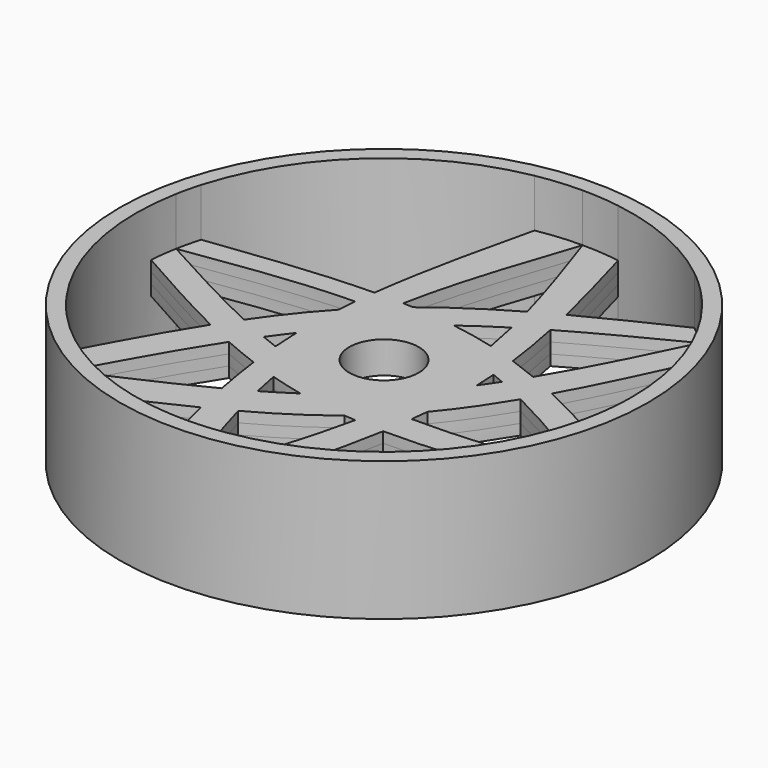
from build123d import *

# Parameters (mm, degrees)
F0_R          = 241.3141538393
F1_DEPTH      = 63.5
F1_DEPTH_BACK = 63.5
F2_DEPTH      = 9.7028
F2_DEPTH_BACK = 9.7028
F3_DEPTH      = 9.7028
F3_DEPTH_BACK = 9.7028
F4_DEPTH      = 9.7028
F4_DEPTH_BACK = 9.7028
F0_R_2        = 31.7673719728
F5_DEPTH      = 9.7028
F5_DEPTH_BACK = 9.7028
F6_DEPTH      = 9.7028
F6_DEPTH_BACK = 9.7028


# Not quite as in the source:
# - a feature of the source that left no trace in its solid (it failed there, or was rolled back) is left out
# - a feature names something its author has since deleted; it is built from what else it names


with BuildPart() as f1:
    # F0 (on Top) → F1 (new body, two sides)
    with BuildSketch(Plane.XY) as f1_sk:
        Circle(F0_R)
        with BuildLine():
            ThreePointArc((178.3079100104, 140.332604898), (214.4135352432, 74.2548764339), (226.9073616472, 0))
            ThreePointArc((226.9073616472, 0), (226.6842601254, -10.0596710247), (226.0153942788, -20.0995601621))
            ThreePointArc((226.0153942788, -20.0995601621), (224.3142281841, -34.2064000428), (221.733453838, -48.1791056247))
            ThreePointArc((221.733453838, -48.1791056247), (218.4875359512, -61.2384471037), (214.4731856165, -74.0824096614))
            ThreePointArc((214.4731856165, -74.0824096614), (145.4794819638, -174.134060704), (34.7509421656, -224.2305126166))
            ThreePointArc((34.7509421656, -224.2305126166), (17.4269439528, -226.2371596228), (0, -226.9073616472))
            ThreePointArc((0, -226.9073616472), (-17.4269439528, -226.2371596228), (-34.7509421656, -224.2305126166))
            ThreePointArc((-34.7509421656, -224.2305126166), (-90.7197460911, -207.9828801581), (-140.7039473309, -178.0150273859))
            ThreePointArc((-140.7039473309, -178.0150273859), (-153.7906323304, -166.8394203332), (-165.9927059169, -154.704144586))
            ThreePointArc((-165.9927059169, -154.704144586), (-176.0017718986, -143.2142697438), (-185.2170956029, -131.0785194688))
            ThreePointArc((-185.2170956029, -131.0785194688), (-218.634724648, -60.7108552716), (-226.2836655529, 16.8123012599))
            ThreePointArc((-226.2836655529, 16.8123012599), (-225.0281851573, 29.1421799891), (-223.1013732807, 41.3851182186))
            ThreePointArc((-223.1013732807, 41.3851182186), (-220.7427090788, 52.5319632059), (-217.8274802779, 63.5463579248))
            ThreePointArc((-217.8274802779, 63.5463579248), (-152.0556560856, 168.4221725964), (-41.0251201184, 223.1678522749))
            ThreePointArc((-41.0251201184, 223.1678522749), (-20.5975994419, 225.9705504417), (0, 226.9073616472))
            ThreePointArc((0, 226.9073616472), (17.325289581, 226.2449670394), (34.5494261777, 224.2616505792))
            ThreePointArc((34.5494261777, 224.2616505792), (91.3796204536, 207.6938028336), (141.9905839779, 176.9904653684))
            ThreePointArc((141.9905839779, 176.9904653684), (151.0506346969, 169.324116792), (159.6974427922, 161.1945332055))
            ThreePointArc((159.6974427922, 161.1945332055), (169.3242736408, 151.050458873), (178.3079100104, 140.332604898))
        make_face(mode=Mode.SUBTRACT)
    extrude(amount=F1_DEPTH)
    extrude(f1_sk.sketch, amount=-F1_DEPTH_BACK)

    # F0 (on Top) → F2 (join, two sides)
    with BuildSketch(Plane.XY) as f2_sk:
        with BuildLine():
            add(Edge.make_bspline(
                [(-223.1013732807, 41.3851182186), (-187.7970771474, 22.1615793919), (-152.5240311166, 2.6878342087), (-116.7614189474, -13.841576746)],
                knots=[0, 0, 0, 0, 0.2511601881, 0.2511601881, 0.2511601881, 0.2511601881], degree=3))
            ThreePointArc((-223.1013732807, 41.3851182186), (-225.0281851573, 29.1421799891), (-226.2836655529, 16.8123012599))
            add(Edge.make_bspline(
                [(-226.2836655529, 16.8123012599), (-194.4717454799, -1.1394771145), (-162.6487337642, -19.090575894), (-130.5710356825, -34.8135274055)],
                knots=[0, 0, 0, 0, 0.2250871065, 0.2250871065, 0.2250871065, 0.2250871065], degree=3))
            add(Edge.make_bspline(
                [(-116.7614189474, -13.841576746), (-121.4836444158, -20.7174022597), (-126.0789503614, -27.7156968125), (-130.5710356828, -34.8135274064)],
                knots=[0.7062454841, 0.7062454841, 0.7062454841, 0.7062454841, 0.7612094599, 0.7612094599, 0.7612094599, 0.7612094599], degree=3))
        make_face()
        with BuildLine():
            ThreePointArc((-185.2170956029, -131.0785194688), (-176.0017718986, -143.2142697438), (-165.9927059169, -154.704144586))
            add(Edge.make_bspline(
                [(-103.8007523743, -47.3412327817), (-126.030548472, -81.5945859435), (-145.9101294083, -118.2760524876), (-165.9927059169, -154.704144586)],
                knots=[0.7370824764, 0.7370824764, 0.7370824764, 0.7370824764, 1, 1, 1, 1], degree=3))
            add(Edge.make_bspline(
                [(-130.5710356825, -34.8135274055), (-121.6689580768, -39.1768995586), (-112.7472657537, -43.3686705384), (-103.8007523743, -47.3412327817)],
                knots=[0.2250871065, 0.2250871065, 0.2250871065, 0.2250871065, 0.2875524021, 0.2875524021, 0.2875524021, 0.2875524021], degree=3))
            add(Edge.make_bspline(
                [(-130.5710356828, -34.8135274064), (-150.0868633876, -65.6499939995), (-167.6544421985, -98.3651644216), (-185.2170956029, -131.0785194688)],
                knots=[0.7612094599, 0.7612094599, 0.7612094599, 0.7612094599, 1, 1, 1, 1], degree=3))
        make_face()
        with BuildLine():
            add(Edge.make_bspline(
                [(-116.7614189474, -13.841576746), (-107.6387205848, -18.0580704836), (-98.4841656138, -22.0829731469), (-89.2891089992, -25.8632585175)],
                knots=[0.2511601881, 0.2511601881, 0.2511601881, 0.2511601881, 0.3152287362, 0.3152287362, 0.3152287362, 0.3152287362], degree=3))
            add(Edge.make_bspline(
                [(-116.7614189474, -13.841576746), (-121.4836444158, -20.7174022597), (-126.0789503614, -27.7156968125), (-130.5710356828, -34.8135274064)],
                knots=[0.7062454841, 0.7062454841, 0.7062454841, 0.7062454841, 0.7612094599, 0.7612094599, 0.7612094599, 0.7612094599], degree=3))
            add(Edge.make_bspline(
                [(-130.5710356825, -34.8135274055), (-121.6689580768, -39.1768995586), (-112.7472657537, -43.3686705384), (-103.8007523743, -47.3412327817)],
                knots=[0.2250871065, 0.2250871065, 0.2250871065, 0.2250871065, 0.2875524021, 0.2875524021, 0.2875524021, 0.2875524021], degree=3))
            add(Edge.make_bspline(
                [(-89.2891089992, -25.8632585175), (-94.2487356362, -32.8958346395), (-99.0777879744, -40.0637315915), (-103.8007523743, -47.3412327817)],
                knots=[0.6812227601, 0.6812227601, 0.6812227601, 0.6812227601, 0.7370824764, 0.7370824764, 0.7370824764, 0.7370824764], degree=3))
        make_face()
        with BuildLine():
            ThreePointArc((-165.9927059169, -154.704144586), (-153.7906323304, -166.8394203332), (-140.7039473309, -178.0150273859))
            add(Edge.make_bspline(
                [(-56.1350371859, -138.940325702), (-83.5712231498, -152.586887822), (-112.1740051357, -165.0586791026), (-140.7039473309, -178.0150273859)],
                knots=[0.8020879998, 0.8020879998, 0.8020879998, 0.8020879998, 1, 1, 1, 1], degree=3))
            add(Edge.make_bspline(
                [(-62.9704662026, -106.5559716315), (-60.8774510593, -117.3512347545), (-58.580284651, -128.146141133), (-56.1350371658, -138.9403257269)],
                knots=[0.7369714232, 0.7369714232, 0.7369714232, 0.7369714232, 0.8093413391, 0.8093413391, 0.8093413391, 0.8093413391], degree=3))
            add(Edge.make_bspline(
                [(-62.9704662042, -106.5559716298), (-95.7578523664, -123.7944289451), (-130.7016529053, -138.8997980839), (-165.9927059169, -154.704144586)],
                knots=[0.7607464131, 0.7607464131, 0.7607464131, 0.7607464131, 1, 1, 1, 1], degree=3))
        make_face()
        with BuildLine():
            add(Edge.make_bspline(
                [(-32.0325540387, -126.4279660664), (-39.9421861303, -130.7313342854), (-47.9871680873, -134.8876340507), (-56.1350371859, -138.940325702)],
                knots=[0.7433130275, 0.7433130275, 0.7433130275, 0.7433130275, 0.8020879998, 0.8020879998, 0.8020879998, 0.8020879998], degree=3))
            add(Edge.make_bspline(
                [(-40.265203536, -94.0296077094), (-37.8015476904, -104.8290604959), (-35.0304565905, -115.6285132824), (-32.0325540365, -126.427966069)],
                knots=[0.7071982306, 0.7071982306, 0.7071982306, 0.7071982306, 0.7785893881, 0.7785893881, 0.7785893881, 0.7785893881], degree=3))
            add(Edge.make_bspline(
                [(-40.2652035459, -94.0296076995), (-47.6992550372, -98.3469624252), (-55.2754717241, -102.5102135071), (-62.9704662042, -106.5559716298)],
                knots=[0.7045950925, 0.7045950925, 0.7045950925, 0.7045950925, 0.7607464131, 0.7607464131, 0.7607464131, 0.7607464131], degree=3))
            add(Edge.make_bspline(
                [(-62.9704662026, -106.5559716315), (-60.8774510593, -117.3512347545), (-58.580284651, -128.146141133), (-56.1350371658, -138.9403257269)],
                knots=[0.7369714232, 0.7369714232, 0.7369714232, 0.7369714232, 0.8093413391, 0.8093413391, 0.8093413391, 0.8093413391], degree=3))
        make_face()
        with BuildLine():
            ThreePointArc((-34.7509421656, -224.2305126166), (-17.4269439528, -226.2371596228), (0, -226.9073616472))
            add(Edge.make_bspline(
                [(-32.0325540365, -126.427966069), (-22.73493984, -159.9210979284), (-11.2557363122, -193.4142297878), (0, -226.9073616472)],
                knots=[0.7785893881, 0.7785893881, 0.7785893881, 0.7785893881, 1, 1, 1, 1], degree=3))
            add(Edge.make_bspline(
                [(-32.0325540387, -126.4279660664), (-39.9421861303, -130.7313342854), (-47.9871680873, -134.8876340507), (-56.1350371859, -138.940325702)],
                knots=[0.7433130275, 0.7433130275, 0.7433130275, 0.7433130275, 0.8020879998, 0.8020879998, 0.8020879998, 0.8020879998], degree=3))
            add(Edge.make_bspline(
                [(-56.1350371658, -138.9403257269), (-49.6930286967, -167.3776225623), (-42.2232488822, -195.8099097806), (-34.7509421656, -224.2305126166)],
                knots=[0.8093413391, 0.8093413391, 0.8093413391, 0.8093413391, 1, 1, 1, 1], degree=3))
        make_face()
        with BuildLine():
            add(Edge.make_bspline(
                [(60.3659257227, -58.8348088049), (58.4669517744, -60.8086435456), (53.2706050834, -66.0612229639), (47.888655793, -71.0891672808), (44.430002216, -74.1731903463)],
                knots=[0.4891405798, 0.4891405798, 0.4891405798, 0.4891405798, 0.5073244479, 0.538264786, 0.538264786, 0.538264786, 0.538264786], degree=3))
            add(Edge.make_bspline(
                [(47.1955269779, -58.2406767098), (51.5760143789, -58.4979061921), (55.9664240103, -58.6943119153), (60.3659257288, -58.8348088167)],
                knots=[0.6237120641, 0.6237120641, 0.6237120641, 0.6237120641, 0.6525763095, 0.6525763095, 0.6525763095, 0.6525763095], degree=3))
            add(Edge.make_bspline(
                [(47.1955269766, -58.2406767095), (46.366376749, -63.5515145884), (45.4413390214, -68.8623524674), (44.430002216, -74.1731903463)],
                knots=[0.6283358025, 0.6283358025, 0.6283358025, 0.6283358025, 0.6634437724, 0.6634437724, 0.6634437724, 0.6634437724], degree=3))
        make_face()
        with BuildLine():
            ThreePointArc((221.733453838, -48.1791056247), (224.3142281841, -34.2064000428), (226.0153942788, -20.0995601621))
            add(Edge.make_bspline(
                [(126.0994867384, 34.1240947789), (160.0186435325, 18.0746130851), (193.0176522959, -1.0122474443), (226.0153942788, -20.0995601621)],
                knots=[0.752086296, 0.752086296, 0.752086296, 0.752086296, 1, 1, 1, 1], degree=3))
            add(Edge.make_bspline(
                [(126.0994867384, 34.1240947789), (122.2078656767, 27.0773550144), (118.2234112411, 20.1283415728), (114.1265769663, 13.3035078657)],
                knots=[0.2438163692, 0.2438163692, 0.2438163692, 0.2438163692, 0.2941816592, 0.2941816592, 0.2941816592, 0.2941816592], degree=3))
            add(Edge.make_bspline(
                [(114.1265769663, 13.3035078657), (150.4723295891, -4.8167201502), (186.0717619128, -26.6529777366), (221.733453838, -48.1791056247)],
                knots=[0.7408189422, 0.7408189422, 0.7408189422, 0.7408189422, 1, 1, 1, 1], degree=3))
        make_face()
        with BuildLine():
            add(Edge.make_bspline(
                [(178.3079100104, 140.332604898), (161.6023122909, 104.6402758365), (144.938669773, 68.2370821736), (126.0994867384, 34.1240947789)],
                knots=[0, 0, 0, 0, 0.2438163692, 0.2438163692, 0.2438163692, 0.2438163692], degree=3))
            ThreePointArc((178.3079100104, 140.332604898), (169.3242736408, 151.050458873), (159.6974427922, 161.1945332055))
            add(Edge.make_bspline(
                [(159.6974427922, 161.1945332055), (140.9740911957, 122.2693377019), (121.7499787846, 82.5474043001), (99.532388565, 45.9349903922)],
                knots=[0, 0, 0, 0, 0.2691785702, 0.2691785702, 0.2691785702, 0.2691785702], degree=3))
            add(Edge.make_bspline(
                [(99.5323885815, 45.9349903786), (108.4605180487, 42.2371577797), (117.3108894654, 38.2825835027), (126.0994867384, 34.1240947789)],
                knots=[0.6878508047, 0.6878508047, 0.6878508047, 0.6878508047, 0.752086296, 0.752086296, 0.752086296, 0.752086296], degree=3))
        make_face()
        with BuildLine():
            add(Edge.make_bspline(
                [(126.0994867384, 34.1240947789), (122.2078656767, 27.0773550144), (118.2234112411, 20.1283415728), (114.1265769663, 13.3035078657)],
                knots=[0.2438163692, 0.2438163692, 0.2438163692, 0.2438163692, 0.2941816592, 0.2941816592, 0.2941816592, 0.2941816592], degree=3))
            add(Edge.make_bspline(
                [(99.5323885815, 45.9349903786), (108.4605180487, 42.2371577797), (117.3108894654, 38.2825835027), (126.0994867384, 34.1240947789)],
                knots=[0.6878508047, 0.6878508047, 0.6878508047, 0.6878508047, 0.752086296, 0.752086296, 0.752086296, 0.752086296], degree=3))
            add(Edge.make_bspline(
                [(99.532388565, 45.9349903922), (95.4389768508, 39.1894485718), (91.243951266, 32.5494596673), (86.9317220877, 26.0394538371)],
                knots=[0.2691785702, 0.2691785702, 0.2691785702, 0.2691785702, 0.3187725497, 0.3187725497, 0.3187725497, 0.3187725497], degree=3))
            add(Edge.make_bspline(
                [(86.9317220877, 26.0394538371), (96.0508128029, 22.0637056796), (105.1116517287, 17.797912), (114.1265769663, 13.3035078657)],
                knots=[0.6765336354, 0.6765336354, 0.6765336354, 0.6765336354, 0.7408189422, 0.7408189422, 0.7408189422, 0.7408189422], degree=3))
        make_face()
        with BuildLine():
            add(Edge.make_bspline(
                [(72.5248897002, -59.0843860265), (71.3623043995, -68.1985786181), (69.9708126845, -77.3125549008), (68.3882994897, -86.4263567185)],
                knots=[0.6317623147, 0.6317623147, 0.6317623147, 0.6317623147, 0.6927246064, 0.6927246064, 0.6927246064, 0.6927246064], degree=3))
            add(Edge.make_bspline(
                [(60.3659257288, -58.8348088167), (64.4114410305, -58.9640012573), (68.4646441716, -59.045919839), (72.5248896994, -59.0843860194)],
                knots=[0.6525763095, 0.6525763095, 0.6525763095, 0.6525763095, 0.6791181212, 0.6791181212, 0.6791181212, 0.6791181212], degree=3))
            add(Edge.make_bspline(
                [(60.3659257227, -58.8348088049), (58.4669517744, -60.8086435456), (53.2706050834, -66.0612229639), (47.888655793, -71.0891672808), (44.430002216, -74.1731903463)],
                knots=[0.4891405798, 0.4891405798, 0.4891405798, 0.4891405798, 0.5073244479, 0.538264786, 0.538264786, 0.538264786, 0.538264786], degree=3))
            add(Edge.make_bspline(
                [(44.430002216, -74.1731903463), (43.7097214036, -77.9556044756), (42.9456663908, -81.7380186049), (42.1413010769, -85.5204327342)],
                knots=[0.6634437724, 0.6634437724, 0.6634437724, 0.6634437724, 0.6884479025, 0.6884479025, 0.6884479025, 0.6884479025], degree=3))
            add(Edge.make_bspline(
                [(42.1413010837, -85.5204327366), (50.8627373609, -86.0716670947), (59.6132744903, -86.3601778015), (68.3882994892, -86.4263567151)],
                knots=[0.6205920902, 0.6205920902, 0.6205920902, 0.6205920902, 0.6790156356, 0.6790156356, 0.6790156356, 0.6790156356], degree=3))
        make_face()
        with BuildLine():
            ThreePointArc((0, -226.9073616472), (17.4269439528, -226.2371596228), (34.7509421656, -224.2305126166))
            add(Edge.make_bspline(
                [(68.3882994897, -86.4263567185), (60.4117725039, -132.36372165), (47.5821906288, -178.2966541593), (34.7509421656, -224.2305126166)],
                knots=[0.6927246064, 0.6927246064, 0.6927246064, 0.6927246064, 1, 1, 1, 1], degree=3))
            add(Edge.make_bspline(
                [(42.1413010837, -85.5204327366), (50.8627373609, -86.0716670947), (59.6132744903, -86.3601778015), (68.3882994892, -86.4263567151)],
                knots=[0.6205920902, 0.6205920902, 0.6205920902, 0.6205920902, 0.6790156356, 0.6790156356, 0.6790156356, 0.6790156356], degree=3))
            add(Edge.make_bspline(
                [(42.1413010769, -85.5204327342), (32.1188887968, -132.6494090385), (15.8382122093, -179.7783853429), (0, -226.9073616472)],
                knots=[0.6884479025, 0.6884479025, 0.6884479025, 0.6884479025, 1, 1, 1, 1], degree=3))
        make_face()
        with BuildLine():
            ThreePointArc((214.4731856165, -74.0824096614), (218.4875359512, -61.2384471037), (221.733453838, -48.1791056247))
            add(Edge.make_bspline(
                [(72.5248896994, -59.0843860194), (121.6119386909, -59.5494296394), (171.7283046479, -53.663459736), (221.733453838, -48.1791056247)],
                knots=[0.6791181212, 0.6791181212, 0.6791181212, 0.6791181212, 1, 1, 1, 1], degree=3))
            add(Edge.make_bspline(
                [(72.5248897002, -59.0843860265), (71.3623043995, -68.1985786181), (69.9708126845, -77.3125549008), (68.3882994897, -86.4263567185)],
                knots=[0.6317623147, 0.6317623147, 0.6317623147, 0.6317623147, 0.6927246064, 0.6927246064, 0.6927246064, 0.6927246064], degree=3))
            add(Edge.make_bspline(
                [(68.3882994892, -86.4263567151), (116.5990987769, -86.78994979), (165.5490656943, -80.4424459657), (214.4731856165, -74.0824096614)],
                knots=[0.6790156356, 0.6790156356, 0.6790156356, 0.6790156356, 1, 1, 1, 1], degree=3))
        make_face()
        with BuildLine():
            add(Edge.make_bspline(
                [(159.6974427922, 161.1945332055), (127.3125749824, 144.6273798519), (94.7583746465, 128.244400412), (63.7576337395, 110.2475227747)],
                knots=[0, 0, 0, 0, 0.2302122603, 0.2302122603, 0.2302122603, 0.2302122603], degree=3))
            ThreePointArc((159.6974427922, 161.1945332055), (151.0506346969, 169.324116792), (141.9905839779, 176.9904653684))
            add(Edge.make_bspline(
                [(141.9905839779, 176.9904653684), (113.68205818, 163.5520272179), (85.3664258812, 150.1027410092), (58.1058267487, 135.6234119333)],
                knots=[0, 0, 0, 0, 0.1962065387, 0.1962065387, 0.1962065387, 0.1962065387], degree=3))
            add(Edge.make_bspline(
                [(58.1058267487, 135.6234119333), (60.1058254664, 127.1652640639), (61.9998462927, 118.7065847162), (63.7576337353, 110.2475227788)],
                knots=[0.1976919219, 0.1976919219, 0.1976919219, 0.1976919219, 0.2542686524, 0.2542686524, 0.2542686524, 0.2542686524], degree=3))
        make_face()
        with BuildLine():
            add(Edge.make_bspline(
                [(63.7576337395, 110.2475227747), (55.6747712661, 105.5551740553), (47.6975141979, 100.7531112553), (39.8563985376, 95.8094640523)],
                knots=[0.2302122603, 0.2302122603, 0.2302122603, 0.2302122603, 0.2902357948, 0.2902357948, 0.2902357948, 0.2902357948], degree=3))
            add(Edge.make_bspline(
                [(58.1058267487, 135.6234119333), (60.1058254664, 127.1652640639), (61.9998462927, 118.7065847162), (63.7576337353, 110.2475227788)],
                knots=[0.1976919219, 0.1976919219, 0.1976919219, 0.1976919219, 0.2542686524, 0.2542686524, 0.2542686524, 0.2542686524], degree=3))
            add(Edge.make_bspline(
                [(58.1058267487, 135.6234119333), (49.7160303444, 131.1672140915), (41.4261644637, 126.6134527547), (33.2671911565, 121.9324177431)],
                knots=[0.1962065387, 0.1962065387, 0.1962065387, 0.1962065387, 0.2565915987, 0.2565915987, 0.2565915987, 0.2565915987], degree=3))
            add(Edge.make_bspline(
                [(33.2671911878, 121.9324177444), (35.6324108412, 113.2247665132), (37.8429009939, 104.517115282), (39.8563985708, 95.8094640508)],
                knots=[0.2313167434, 0.2313167434, 0.2313167434, 0.2313167434, 0.2888797804, 0.2888797804, 0.2888797804, 0.2888797804], degree=3))
        make_face()
        with BuildLine():
            add(Edge.make_bspline(
                [(34.5494261777, 224.2616505792), (42.8349791403, 194.7262948915), (51.1173778447, 165.1780979869), (58.1058267487, 135.6234119333)],
                knots=[0, 0, 0, 0, 0.1976919219, 0.1976919219, 0.1976919219, 0.1976919219], degree=3))
            ThreePointArc((34.5494261777, 224.2616505792), (17.325289581, 226.2449670394), (0, 226.9073616472))
            add(Edge.make_bspline(
                [(0, 226.9073616472), (11.7593291755, 191.9157136796), (23.7625691856, 156.924065712), (33.2671911878, 121.9324177444)],
                knots=[0, 0, 0, 0, 0.2313167434, 0.2313167434, 0.2313167434, 0.2313167434], degree=3))
            add(Edge.make_bspline(
                [(58.1058267487, 135.6234119333), (49.7160303444, 131.1672140915), (41.4261644637, 126.6134527547), (33.2671911565, 121.9324177431)],
                knots=[0.1962065387, 0.1962065387, 0.1962065387, 0.1962065387, 0.2565915987, 0.2565915987, 0.2565915987, 0.2565915987], degree=3))
        make_face()
        with BuildLine():
            add(Edge.make_bspline(
                [(0, 226.9073616472), (-16.8174769673, 176.8644361569), (-34.1338242703, 126.8215106665), (-43.926978592, 76.7785851761)],
                knots=[0, 0, 0, 0, 0.3308151295, 0.3308151295, 0.3308151295, 0.3308151295], degree=3))
            ThreePointArc((0, 226.9073616472), (-20.5975994419, 225.9705504417), (-41.0251201184, 223.1678522749))
            add(Edge.make_bspline(
                [(-41.0251201184, 223.1678522749), (-52.4783431881, 174.4093664115), (-63.9341990007, 125.6686491297), (-70.1940115867, 76.9227656283)],
                knots=[0, 0, 0, 0, 0.32691305, 0.32691305, 0.32691305, 0.32691305], degree=3))
            add(Edge.make_bspline(
                [(-70.1940115868, 76.9227656286), (-61.379684587, 77.0697268961), (-52.6205760006, 77.0328679317), (-43.926978593, 76.7785851835)],
                knots=[0.3061572354, 0.3061572354, 0.3061572354, 0.3061572354, 0.3622331035, 0.3622331035, 0.3622331035, 0.3622331035], degree=3))
        make_face()
        with BuildLine():
            add(Edge.make_bspline(
                [(-43.926978592, 76.7785851761), (-44.5432752393, 73.6293151671), (-45.1297773513, 70.480045158), (-45.6844855831, 67.330775149)],
                knots=[0.3308151295, 0.3308151295, 0.3308151295, 0.3308151295, 0.3516337798, 0.3516337798, 0.3516337798, 0.3516337798], degree=3))
            add(Edge.make_bspline(
                [(-70.1940115868, 76.9227656286), (-61.379684587, 77.0697268961), (-52.6205760006, 77.0328679317), (-43.926978593, 76.7785851835)],
                knots=[0.3061572354, 0.3061572354, 0.3061572354, 0.3061572354, 0.3622331035, 0.3622331035, 0.3622331035, 0.3622331035], degree=3))
            add(Edge.make_bspline(
                [(-70.1940115867, 76.9227656283), (-71.0199395156, 70.4911694667), (-71.7554120654, 64.0594833688), (-72.3884883871, 57.6276546558)],
                knots=[0.32691305, 0.32691305, 0.32691305, 0.32691305, 0.370046389, 0.370046389, 0.370046389, 0.370046389], degree=3))
            add(Edge.make_bspline(
                [(-72.3884883872, 57.6276546558), (-67.0646442905, 57.7244107708), (-61.7571998837, 57.7395100868), (-56.468043341, 57.6635508246)],
                knots=[0.3185902737, 0.3185902737, 0.3185902737, 0.3185902737, 0.3529732947, 0.3529732947, 0.3529732947, 0.3529732947], degree=3))
            add(Edge.make_bspline(
                [(-45.6844855556, 67.3307751349), (-49.3482288534, 64.1752671457), (-52.9443087815, 60.9543566074), (-56.4680433413, 57.6635508256)],
                knots=[0.4662407645, 0.4662407645, 0.4662407645, 0.4662407645, 0.4984116757, 0.4984116757, 0.4984116757, 0.4984116757], degree=3))
        make_face()
        with BuildLine():
            add(Edge.make_bspline(
                [(-217.8274802779, 63.5463579248), (-168.0870830213, 69.8386711876), (-118.3175641023, 76.1204016734), (-70.1940115868, 76.9227656286)],
                knots=[0, 0, 0, 0, 0.3061572354, 0.3061572354, 0.3061572354, 0.3061572354], degree=3))
            ThreePointArc((-217.8274802779, 63.5463579248), (-220.7427090788, 52.5319632059), (-223.1013732807, 41.3851182186))
            add(Edge.make_bspline(
                [(-223.1013732807, 41.3851182186), (-172.457132659, 48.8237580971), (-121.7187944055, 56.7311203711), (-72.3884883872, 57.6276546558)],
                knots=[0, 0, 0, 0, 0.3185902737, 0.3185902737, 0.3185902737, 0.3185902737], degree=3))
            add(Edge.make_bspline(
                [(-70.1940115867, 76.9227656283), (-71.0199395156, 70.4911694667), (-71.7554120654, 64.0594833688), (-72.3884883871, 57.6276546558)],
                knots=[0.32691305, 0.32691305, 0.32691305, 0.32691305, 0.370046389, 0.370046389, 0.370046389, 0.370046389], degree=3))
        make_face()
        with BuildLine():
            add(Edge.make_bspline(
                [(-45.6844855831, 67.330775149), (-46.2652649637, 64.0334902339), (-46.8111916233, 60.7362053189), (-47.3199708539, 57.4389204039)],
                knots=[0.3516337798, 0.3516337798, 0.3516337798, 0.3516337798, 0.3734309015, 0.3734309015, 0.3734309015, 0.3734309015], degree=3))
            add(Edge.make_bspline(
                [(-45.6844855556, 67.3307751349), (-49.3482288534, 64.1752671457), (-52.9443087815, 60.9543566074), (-56.4680433413, 57.6635508256)],
                knots=[0.4662407645, 0.4662407645, 0.4662407645, 0.4662407645, 0.4984116757, 0.4984116757, 0.4984116757, 0.4984116757], degree=3))
            add(Edge.make_bspline(
                [(-56.468043341, 57.6635508246), (-53.412461006, 57.6196686332), (-50.3629821594, 57.5453960707), (-47.3199708543, 57.4389204085)],
                knots=[0.3529732947, 0.3529732947, 0.3529732947, 0.3529732947, 0.3728366038, 0.3728366038, 0.3728366038, 0.3728366038], degree=3))
        make_face()
        with BuildLine():
            add(Edge.make_bspline(
                [(-74.8748334574, -6.3317792212), (-79.8096642217, -12.7072810815), (-84.6075579763, -19.2249838353), (-89.2891089992, -25.8632585175)],
                knots=[0.6284949781, 0.6284949781, 0.6284949781, 0.6284949781, 0.6812227601, 0.6812227601, 0.6812227601, 0.6812227601], degree=3))
            add(Edge.make_bspline(
                [(-73.8401592874, 40.262906217), (-74.7563166341, 26.8429241355), (-75.2465760161, 11.3117584788), (-74.9320157638, -4.2211556835), (-74.8748334608, -6.3317792203)],
                knots=[0.4088628756, 0.4088628756, 0.4088628756, 0.4088628756, 0.4988562077, 0.5130072176, 0.5130072176, 0.5130072176, 0.5130072176], degree=3))
            add(Edge.make_bspline(
                [(-73.8401592874, 40.262906217), (-89.4730644421, 23.5083445643), (-103.6094896571, 5.3083710008), (-116.7614189474, -13.841576746)],
                knots=[0.553164627, 0.553164627, 0.553164627, 0.553164627, 0.7062454841, 0.7062454841, 0.7062454841, 0.7062454841], degree=3))
            add(Edge.make_bspline(
                [(-116.7614189474, -13.841576746), (-107.6387205848, -18.0580704836), (-98.4841656138, -22.0829731469), (-89.2891089992, -25.8632585175)],
                knots=[0.2511601881, 0.2511601881, 0.2511601881, 0.2511601881, 0.3152287362, 0.3152287362, 0.3152287362, 0.3152287362], degree=3))
        make_face()
        with BuildLine():
            add(Edge.make_bspline(
                [(39.8563985376, 95.8094640523), (28.1496006924, 88.4285911089), (16.7462693467, 80.7321189379), (5.7480277227, 72.6139837278)],
                knots=[0.2902357948, 0.2902357948, 0.2902357948, 0.2902357948, 0.3798510249, 0.3798510249, 0.3798510249, 0.3798510249], degree=3))
            add(Edge.make_bspline(
                [(33.2671911878, 121.9324177444), (35.6324108412, 113.2247665132), (37.8429009939, 104.517115282), (39.8563985708, 95.8094640508)],
                knots=[0.2313167434, 0.2313167434, 0.2313167434, 0.2313167434, 0.2888797804, 0.2888797804, 0.2888797804, 0.2888797804], degree=3))
            add(Edge.make_bspline(
                [(33.2671911565, 121.9324177431), (9.2009096149, 108.1249076248), (-13.7265338796, 93.2100458867), (-34.7205364248, 76.425357331)],
                knots=[0.2565915987, 0.2565915987, 0.2565915987, 0.2565915987, 0.4347076189, 0.4347076189, 0.4347076189, 0.4347076189], degree=3))
            add(Edge.make_bspline(
                [(-34.7205364244, 76.4253573294), (-21.0444056104, 75.7730059641), (-7.5413053085, 74.5468801984), (5.7480277227, 72.6139837278)],
                knots=[0.3820816414, 0.3820816414, 0.3820816414, 0.3820816414, 0.4707824274, 0.4707824274, 0.4707824274, 0.4707824274], degree=3))
        make_face()
        with BuildLine():
            add(Edge.make_bspline(
                [(-40.265203536, -94.0296077094), (-37.8015476904, -104.8290604959), (-35.0304565905, -115.6285132824), (-32.0325540365, -126.427966069)],
                knots=[0.7071982306, 0.7071982306, 0.7071982306, 0.7071982306, 0.7785893881, 0.7785893881, 0.7785893881, 0.7785893881], degree=3))
            add(Edge.make_bspline(
                [(31.9130911216, -84.7499075032), (12.2215313381, -100.5355617573), (-9.3489145049, -114.0865508996), (-32.0325540387, -126.4279660664)],
                knots=[0.5747552146, 0.5747552146, 0.5747552146, 0.5747552146, 0.7433130275, 0.7433130275, 0.7433130275, 0.7433130275], degree=3))
            add(Edge.make_bspline(
                [(-14.2194983817, -77.7999720616), (-11.9253735013, -78.3022354633), (3.3554365238, -81.4870898234), (18.7563063515, -83.5956084544), (31.9130911219, -84.7499075041)],
                knots=[0.4937168769, 0.4937168769, 0.4937168769, 0.4937168769, 0.5093492669, 0.597722539, 0.597722539, 0.597722539, 0.597722539], degree=3))
            add(Edge.make_bspline(
                [(-14.2194983817, -77.7999720616), (-22.6709402637, -83.4725390625), (-31.3662142842, -88.8614845856), (-40.2652035459, -94.0296076995)],
                knots=[0.6373787168, 0.6373787168, 0.6373787168, 0.6373787168, 0.7045950925, 0.7045950925, 0.7045950925, 0.7045950925], degree=3))
        make_face()
        with BuildLine():
            add(Edge.make_bspline(
                [(114.1265769663, 13.3035078657), (102.0034881539, -6.892101625), (88.8963470271, -26.0003332005), (74.2986728866, -43.3357359438)],
                knots=[0.2941816592, 0.2941816592, 0.2941816592, 0.2941816592, 0.4432193901, 0.4432193901, 0.4432193901, 0.4432193901], degree=3))
            add(Edge.make_bspline(
                [(86.9317220877, 26.0394538371), (96.0508128029, 22.0637056796), (105.1116517287, 17.797912), (114.1265769663, 13.3035078657)],
                knots=[0.6765336354, 0.6765336354, 0.6765336354, 0.6765336354, 0.7408189422, 0.7408189422, 0.7408189422, 0.7408189422], degree=3))
            add(Edge.make_bspline(
                [(86.9317220877, 26.0394538371), (83.4755802865, 20.8218500539), (79.9441514206, 15.6877423806), (76.3294093346, 10.6497083496)],
                knots=[0.3187725497, 0.3187725497, 0.3187725497, 0.3187725497, 0.3585208604, 0.3585208604, 0.3585208604, 0.3585208604], degree=3))
            add(Edge.make_bspline(
                [(76.3294093346, 10.6497083496), (76.4228091123, 7.0997663821), (76.6686957813, -10.8962895344), (75.7033319421, -28.8911499579), (74.2986728866, -43.3357359438)],
                knots=[0.4762959402, 0.4762959402, 0.4762959402, 0.4762959402, 0.5000370192, 0.5966500368, 0.5966500368, 0.5966500368, 0.5966500368], degree=3))
        make_face()
        with BuildLine():
            add(Edge.make_bspline(
                [(63.7576337353, 110.2475227788), (67.5092172163, 92.1936464903), (70.6402460129, 74.1380274734), (72.8565835725, 56.0821131885)],
                knots=[0.2542686524, 0.2542686524, 0.2542686524, 0.2542686524, 0.3750183644, 0.3750183644, 0.3750183644, 0.3750183644], degree=3))
            add(Edge.make_bspline(
                [(63.7576337395, 110.2475227747), (55.6747712661, 105.5551740553), (47.6975141979, 100.7531112553), (39.8563985376, 95.8094640523)],
                knots=[0.2302122603, 0.2302122603, 0.2302122603, 0.2302122603, 0.2902357948, 0.2902357948, 0.2902357948, 0.2902357948], degree=3))
            add(Edge.make_bspline(
                [(39.8563985708, 95.8094640508), (42.2874442267, 85.2960678886), (44.4313233221, 74.7826717265), (46.2136505599, 64.2692755643)],
                knots=[0.2888797804, 0.2888797804, 0.2888797804, 0.2888797804, 0.3583799241, 0.3583799241, 0.3583799241, 0.3583799241], degree=3))
            add(Edge.make_bspline(
                [(46.2136505599, 64.2692755643), (55.1915373321, 61.8602745475), (64.0677105755, 59.1153416619), (72.8565835745, 56.0821131912)],
                knots=[0.5623988795, 0.5623988795, 0.5623988795, 0.5623988795, 0.6244574438, 0.6244574438, 0.6244574438, 0.6244574438], degree=3))
        make_face()
        with BuildLine():
            add(Edge.make_bspline(
                [(-40.2652035459, -94.0296076995), (-47.6992550372, -98.3469624252), (-55.2754717241, -102.5102135071), (-62.9704662042, -106.5559716298)],
                knots=[0.7045950925, 0.7045950925, 0.7045950925, 0.7045950925, 0.7607464131, 0.7607464131, 0.7607464131, 0.7607464131], degree=3))
            add(Edge.make_bspline(
                [(-45.282922279, -69.5800492168), (-43.8085348876, -77.7299020476), (-42.1244118649, -85.8797548785), (-40.265203536, -94.0296077094)],
                knots=[0.653322591, 0.653322591, 0.653322591, 0.653322591, 0.7071982306, 0.7071982306, 0.7071982306, 0.7071982306], degree=3))
            add(Edge.make_bspline(
                [(-70.4345665727, -61.0026125154), (-62.0789232061, -64.1133073799), (-53.6964231494, -66.9850844484), (-45.282922279, -69.5800492168)],
                knots=[0.3649186891, 0.3649186891, 0.3649186891, 0.3649186891, 0.4228089569, 0.4228089569, 0.4228089569, 0.4228089569], degree=3))
            add(Edge.make_bspline(
                [(-70.4345665657, -61.0026125069), (-68.4544405797, -76.1870941285), (-65.9143983038, -91.371885769), (-62.9704662026, -106.5559716315)],
                knots=[0.6351794609, 0.6351794609, 0.6351794609, 0.6351794609, 0.7369714232, 0.7369714232, 0.7369714232, 0.7369714232], degree=3))
        make_face()
        with BuildLine():
            add(Edge.make_bspline(
                [(-73.4881541081, -32.0929897185), (-72.7224001604, -41.7292326761), (-71.6912432322, -51.3658601577), (-70.4345665657, -61.0026125069)],
                knots=[0.570577721, 0.570577721, 0.570577721, 0.570577721, 0.6351794609, 0.6351794609, 0.6351794609, 0.6351794609], degree=3))
            add(Edge.make_bspline(
                [(-89.2891089992, -25.8632585175), (-84.0358809303, -28.0229734654), (-78.7694333213, -30.1028465153), (-73.4881541081, -32.0929897185)],
                knots=[0.3152287362, 0.3152287362, 0.3152287362, 0.3152287362, 0.3518317403, 0.3518317403, 0.3518317403, 0.3518317403], degree=3))
            add(Edge.make_bspline(
                [(-89.2891089992, -25.8632585175), (-94.2487356362, -32.8958346395), (-99.0777879744, -40.0637315915), (-103.8007523743, -47.3412327817)],
                knots=[0.6812227601, 0.6812227601, 0.6812227601, 0.6812227601, 0.7370824764, 0.7370824764, 0.7370824764, 0.7370824764], degree=3))
            add(Edge.make_bspline(
                [(-103.8007523743, -47.3412327817), (-92.720063225, -52.2614430892), (-81.6012985272, -56.8453867675), (-70.4345665727, -61.0026125154)],
                knots=[0.2875524021, 0.2875524021, 0.2875524021, 0.2875524021, 0.3649186891, 0.3649186891, 0.3649186891, 0.3649186891], degree=3))
        make_face()
        with BuildLine():
            add(Edge.make_bspline(
                [(99.532388565, 45.9349903922), (95.4389768508, 39.1894485718), (91.243951266, 32.5494596673), (86.9317220877, 26.0394538371)],
                knots=[0.2691785702, 0.2691785702, 0.2691785702, 0.2691785702, 0.3187725497, 0.3187725497, 0.3187725497, 0.3187725497], degree=3))
            add(Edge.make_bspline(
                [(72.8565835745, 56.0821131912), (81.8344934769, 52.983644033), (90.7213073249, 49.5843442126), (99.5323885815, 45.9349903786)],
                knots=[0.6244574438, 0.6244574438, 0.6244574438, 0.6244574438, 0.6878508047, 0.6878508047, 0.6878508047, 0.6878508047], degree=3))
            add(Edge.make_bspline(
                [(72.8565835725, 56.0821131885), (73.8858717177, 47.6967756554), (74.7178827755, 39.31137444), (75.3231554266, 30.926054523)],
                knots=[0.3750183644, 0.3750183644, 0.3750183644, 0.3750183644, 0.4310956739, 0.4310956739, 0.4310956739, 0.4310956739], degree=3))
            add(Edge.make_bspline(
                [(75.3231554265, 30.926054523), (79.20373141, 29.3522262649), (83.0729420123, 27.7218077311), (86.9317220877, 26.0394538371)],
                knots=[0.6493310481, 0.6493310481, 0.6493310481, 0.6493310481, 0.6765336354, 0.6765336354, 0.6765336354, 0.6765336354], degree=3))
        make_face()
        with BuildLine():
            add(Edge.make_bspline(
                [(-72.3884883872, 57.6276546558), (-67.0646442905, 57.7244107708), (-61.7571998837, 57.7395100868), (-56.468043341, 57.6635508246)],
                knots=[0.3185902737, 0.3185902737, 0.3185902737, 0.3185902737, 0.3529732947, 0.3529732947, 0.3529732947, 0.3529732947], degree=3))
            add(Edge.make_bspline(
                [(-72.3884883871, 57.6276546558), (-72.9582054354, 51.8395334711), (-73.4449965729, 46.051296789), (-73.8401592874, 40.262906217)],
                knots=[0.370046389, 0.370046389, 0.370046389, 0.370046389, 0.4088628756, 0.4088628756, 0.4088628756, 0.4088628756], degree=3))
            add(Edge.make_bspline(
                [(-56.4680433413, 57.6635508256), (-57.1536029669, 57.0233086218), (-63.1268317058, 51.3994118216), (-68.8878664111, 45.5705246986), (-73.8401592874, 40.262906217)],
                knots=[0.4984116757, 0.4984116757, 0.4984116757, 0.4984116757, 0.5046706823, 0.553164627, 0.553164627, 0.553164627, 0.553164627], degree=3))
        make_face()
        with BuildLine():
            add(Edge.make_bspline(
                [(-43.926978593, 76.7785851835), (-40.8498047075, 76.6885796087), (-37.7808385026, 76.5713337219), (-34.7205364244, 76.4253573294)],
                knots=[0.3622331035, 0.3622331035, 0.3622331035, 0.3622331035, 0.3820816414, 0.3820816414, 0.3820816414, 0.3820816414], degree=3))
            add(Edge.make_bspline(
                [(-43.926978592, 76.7785851761), (-44.5432752393, 73.6293151671), (-45.1297773513, 70.480045158), (-45.6844855831, 67.330775149)],
                knots=[0.3308151295, 0.3308151295, 0.3308151295, 0.3308151295, 0.3516337798, 0.3516337798, 0.3516337798, 0.3516337798], degree=3))
            add(Edge.make_bspline(
                [(-34.7205364248, 76.425357331), (-38.4372539863, 73.453844558), (-42.0933733733, 70.4237274135), (-45.6844855556, 67.3307751349)],
                knots=[0.4347076189, 0.4347076189, 0.4347076189, 0.4347076189, 0.4662407645, 0.4662407645, 0.4662407645, 0.4662407645], degree=3))
        make_face()
        with BuildLine():
            add(Edge.make_bspline(
                [(31.9130911219, -84.7499075041), (35.3178509045, -85.0486211375), (38.7273464546, -85.3046553087), (42.1413010837, -85.5204327366)],
                knots=[0.597722539, 0.597722539, 0.597722539, 0.597722539, 0.6205920902, 0.6205920902, 0.6205920902, 0.6205920902], degree=3))
            add(Edge.make_bspline(
                [(44.430002216, -74.1731903463), (43.7097214036, -77.9556044756), (42.9456663908, -81.7380186049), (42.1413010769, -85.5204327342)],
                knots=[0.6634437724, 0.6634437724, 0.6634437724, 0.6634437724, 0.6884479025, 0.6884479025, 0.6884479025, 0.6884479025], degree=3))
            add(Edge.make_bspline(
                [(44.430002216, -74.1731903463), (40.3509339395, -77.8104267362), (36.1760406973, -81.3325323005), (31.9130911216, -84.7499075032)],
                knots=[0.538264786, 0.538264786, 0.538264786, 0.538264786, 0.5747552146, 0.5747552146, 0.5747552146, 0.5747552146], degree=3))
        make_face()
        with BuildLine():
            add(Edge.make_bspline(
                [(60.3659257288, -58.8348088167), (64.4114410305, -58.9640012573), (68.4646441716, -59.045919839), (72.5248896994, -59.0843860194)],
                knots=[0.6525763095, 0.6525763095, 0.6525763095, 0.6525763095, 0.6791181212, 0.6791181212, 0.6791181212, 0.6791181212], degree=3))
            add(Edge.make_bspline(
                [(74.2986728866, -43.3357359438), (73.788174609, -48.5853630594), (73.1945006518, -53.8349104219), (72.5248897002, -59.0843860265)],
                knots=[0.5966500368, 0.5966500368, 0.5966500368, 0.5966500368, 0.6317623147, 0.6317623147, 0.6317623147, 0.6317623147], degree=3))
            add(Edge.make_bspline(
                [(74.2986728866, -43.3357359438), (69.8008684792, -48.6770834839), (65.1615578938, -53.8501246328), (60.3659257227, -58.8348088049)],
                knots=[0.4432193901, 0.4432193901, 0.4432193901, 0.4432193901, 0.4891405798, 0.4891405798, 0.4891405798, 0.4891405798], degree=3))
        make_face()
    extrude(amount=F2_DEPTH)
    extrude(f2_sk.sketch, amount=-F2_DEPTH_BACK)

    # F0 (on Top) → F2, piece 2 (join, two sides)
    with BuildSketch(Plane.XY) as f2_2_sk:
        with BuildLine():
            add(Edge.make_bspline(
                [(15.994177773, -55.2903259997), (6.3480987535, -63.3085225022), (-3.7485580572, -70.7719274531), (-14.2194983817, -77.7999720616)],
                knots=[0.554100778, 0.554100778, 0.554100778, 0.554100778, 0.6373787168, 0.6373787168, 0.6373787168, 0.6373787168], degree=3))
            add(Edge.make_bspline(
                [(-49.6052252782, -40.4132889191), (-35.51325606, -44.9045731385), (-13.7769520223, -50.6552663039), (8.311170121, -54.2683340591), (15.9941777688, -55.2903259887)],
                knots=[0.4067628451, 0.4067628451, 0.4067628451, 0.4067628451, 0.5035478242, 0.5547829392, 0.5547829392, 0.5547829392, 0.5547829392], degree=3))
            add(Edge.make_bspline(
                [(-49.6052253017, -40.4132889297), (-48.5021480506, -50.1355423587), (-47.0417721834, -59.8577957877), (-45.282922279, -69.5800492168)],
                knots=[0.5890523971, 0.5890523971, 0.5890523971, 0.5890523971, 0.653322591, 0.653322591, 0.653322591, 0.653322591], degree=3))
            add(Edge.make_bspline(
                [(-45.282922279, -69.5800492168), (-34.9774967065, -72.7585377789), (-24.6255605847, -75.5217245937), (-14.2194983817, -77.7999720616)],
                knots=[0.4228089569, 0.4228089569, 0.4228089569, 0.4228089569, 0.4937168769, 0.4937168769, 0.4937168769, 0.4937168769], degree=3))
        make_face()
    extrude(amount=F2_DEPTH)
    extrude(f2_2_sk.sketch, amount=-F2_DEPTH_BACK)

    # F0 (on Top) → F2, piece 3 (join, two sides)
    with BuildSketch(Plane.XY) as f2_3_sk:
        with BuildLine():
            add(Edge.make_bspline(
                [(15.9941777688, -55.2903259887), (26.3305065582, -56.6652620929), (36.7347247171, -57.626401059), (47.1955269779, -58.2406767098)],
                knots=[0.5547829392, 0.5547829392, 0.5547829392, 0.5547829392, 0.6237120641, 0.6237120641, 0.6237120641, 0.6237120641], degree=3))
            add(Edge.make_bspline(
                [(51.3212515182, -20.9088102779), (50.5546869972, -33.3527657551), (49.1383293652, -45.7967212323), (47.1955269766, -58.2406767095)],
                knots=[0.5460734507, 0.5460734507, 0.5460734507, 0.5460734507, 0.6283358025, 0.6283358025, 0.6283358025, 0.6283358025], degree=3))
            add(Edge.make_bspline(
                [(51.3212515182, -20.9088102779), (45.3051450655, -27.7329701051), (33.914203461, -39.6800411725), (21.6803851525, -50.5637290031), (15.994177773, -55.2903259997)],
                knots=[0.4454913911, 0.4454913911, 0.4454913911, 0.4454913911, 0.5050097816, 0.554100778, 0.554100778, 0.554100778, 0.554100778], degree=3))
        make_face()
    extrude(amount=F2_DEPTH)
    extrude(f2_3_sk.sketch, amount=-F2_DEPTH_BACK)

    # F0 (on Top) → F2, piece 4 (join, two sides)
    with BuildSketch(Plane.XY) as f2_4_sk:
        with BuildLine():
            add(Edge.make_bspline(
                [(75.3231554266, 30.926054523), (75.8110262845, 24.1671943387), (76.1515869684, 17.4083869734), (76.3294093346, 10.6497083496)],
                knots=[0.4310956739, 0.4310956739, 0.4310956739, 0.4310956739, 0.4762959402, 0.4762959402, 0.4762959402, 0.4762959402], degree=3))
            add(Edge.make_bspline(
                [(49.6045199666, 40.4195051352), (58.2387027196, 37.5602673322), (66.8082891483, 34.3793916613), (75.3231554265, 30.926054523)],
                knots=[0.5896423849, 0.5896423849, 0.5896423849, 0.5896423849, 0.6493310481, 0.6493310481, 0.6493310481, 0.6493310481], degree=3))
            add(Edge.make_bspline(
                [(49.6045199682, 40.4195051375), (51.133383371, 26.9463367583), (52.4120219557, 6.5035649532), (51.7505885342, -13.9392068519), (51.3212515182, -20.9088102779)],
                knots=[0.4109339053, 0.4109339053, 0.4109339053, 0.4109339053, 0.5, 0.5460734507, 0.5460734507, 0.5460734507, 0.5460734507], degree=3))
            add(Edge.make_bspline(
                [(76.3294093346, 10.6497083496), (68.4202420907, -0.3736655965), (60.1122145505, -10.9370889927), (51.3212515182, -20.9088102779)],
                knots=[0.3585208604, 0.3585208604, 0.3585208604, 0.3585208604, 0.4454913911, 0.4454913911, 0.4454913911, 0.4454913911], degree=3))
        make_face()
    extrude(amount=F2_DEPTH)
    extrude(f2_4_sk.sketch, amount=-F2_DEPTH_BACK)

    # F0 (on Top) → F3 (join, two sides)
    with BuildSketch(Plane.XY) as f3_sk:
        with BuildLine():
            add(Edge.make_bspline(
                [(-51.2671708451, 21.7699117997), (-59.5036240987, 12.7846051269), (-67.3484915269, 3.391797791), (-74.8748334574, -6.3317792212)],
                knots=[0.5480773639, 0.5480773639, 0.5480773639, 0.5480773639, 0.6284949781, 0.6284949781, 0.6284949781, 0.6284949781], degree=3))
            add(Edge.make_bspline(
                [(-47.3199708539, 57.4389204039), (-49.1545763167, 45.5492508699), (-50.5061726075, 33.659581336), (-51.2671708513, 21.769911802)],
                knots=[0.3734309015, 0.3734309015, 0.3734309015, 0.3734309015, 0.4520290756, 0.4520290756, 0.4520290756, 0.4520290756], degree=3))
            add(Edge.make_bspline(
                [(-56.468043341, 57.6635508246), (-53.412461006, 57.6196686332), (-50.3629821594, 57.5453960707), (-47.3199708543, 57.4389204085)],
                knots=[0.3529732947, 0.3529732947, 0.3529732947, 0.3529732947, 0.3728366038, 0.3728366038, 0.3728366038, 0.3728366038], degree=3))
            add(Edge.make_bspline(
                [(-56.4680433413, 57.6635508256), (-57.1536029669, 57.0233086218), (-63.1268317058, 51.3994118216), (-68.8878664111, 45.5705246986), (-73.8401592874, 40.262906217)],
                knots=[0.4984116757, 0.4984116757, 0.4984116757, 0.4984116757, 0.5046706823, 0.553164627, 0.553164627, 0.553164627, 0.553164627], degree=3))
            add(Edge.make_bspline(
                [(-73.8401592874, 40.262906217), (-74.7563166341, 26.8429241355), (-75.2465760161, 11.3117584788), (-74.9320157638, -4.2211556835), (-74.8748334608, -6.3317792203)],
                knots=[0.4088628756, 0.4088628756, 0.4088628756, 0.4088628756, 0.4988562077, 0.5130072176, 0.5130072176, 0.5130072176, 0.5130072176], degree=3))
        make_face()
    extrude(amount=F3_DEPTH)
    extrude(f3_sk.sketch, amount=-F3_DEPTH_BACK)

    # F0 (on Top) → F4 (join, two sides)
    with BuildSketch(Plane.XY) as f4_sk:
        with BuildLine():
            add(Edge.make_bspline(
                [(72.8565835725, 56.0821131885), (73.8858717177, 47.6967756554), (74.7178827755, 39.31137444), (75.3231554266, 30.926054523)],
                knots=[0.3750183644, 0.3750183644, 0.3750183644, 0.3750183644, 0.4310956739, 0.4310956739, 0.4310956739, 0.4310956739], degree=3))
            add(Edge.make_bspline(
                [(46.2136505599, 64.2692755643), (55.1915373321, 61.8602745475), (64.0677105755, 59.1153416619), (72.8565835745, 56.0821131912)],
                knots=[0.5623988795, 0.5623988795, 0.5623988795, 0.5623988795, 0.6244574438, 0.6244574438, 0.6244574438, 0.6244574438], degree=3))
            add(Edge.make_bspline(
                [(46.2136505599, 64.2692755643), (47.5613944221, 56.3193520887), (48.7024049856, 48.3694286131), (49.6045199682, 40.4195051375)],
                knots=[0.3583799241, 0.3583799241, 0.3583799241, 0.3583799241, 0.4109339053, 0.4109339053, 0.4109339053, 0.4109339053], degree=3))
            add(Edge.make_bspline(
                [(49.6045199666, 40.4195051352), (58.2387027196, 37.5602673322), (66.8082891483, 34.3793916613), (75.3231554265, 30.926054523)],
                knots=[0.5896423849, 0.5896423849, 0.5896423849, 0.5896423849, 0.6493310481, 0.6493310481, 0.6493310481, 0.6493310481], degree=3))
        make_face()
        with BuildLine():
            add(Edge.make_bspline(
                [(75.3231554266, 30.926054523), (75.8110262845, 24.1671943387), (76.1515869684, 17.4083869734), (76.3294093346, 10.6497083496)],
                knots=[0.4310956739, 0.4310956739, 0.4310956739, 0.4310956739, 0.4762959402, 0.4762959402, 0.4762959402, 0.4762959402], degree=3))
            add(Edge.make_bspline(
                [(49.6045199666, 40.4195051352), (58.2387027196, 37.5602673322), (66.8082891483, 34.3793916613), (75.3231554265, 30.926054523)],
                knots=[0.5896423849, 0.5896423849, 0.5896423849, 0.5896423849, 0.6493310481, 0.6493310481, 0.6493310481, 0.6493310481], degree=3))
            add(Edge.make_bspline(
                [(49.6045199682, 40.4195051375), (51.133383371, 26.9463367583), (52.4120219557, 6.5035649532), (51.7505885342, -13.9392068519), (51.3212515182, -20.9088102779)],
                knots=[0.4109339053, 0.4109339053, 0.4109339053, 0.4109339053, 0.5, 0.5460734507, 0.5460734507, 0.5460734507, 0.5460734507], degree=3))
            add(Edge.make_bspline(
                [(76.3294093346, 10.6497083496), (68.4202420907, -0.3736655965), (60.1122145505, -10.9370889927), (51.3212515182, -20.9088102779)],
                knots=[0.3585208604, 0.3585208604, 0.3585208604, 0.3585208604, 0.4454913911, 0.4454913911, 0.4454913911, 0.4454913911], degree=3))
        make_face()
        with BuildLine():
            add(Edge.make_bspline(
                [(74.2986728866, -43.3357359438), (69.8008684792, -48.6770834839), (65.1615578938, -53.8501246328), (60.3659257227, -58.8348088049)],
                knots=[0.4432193901, 0.4432193901, 0.4432193901, 0.4432193901, 0.4891405798, 0.4891405798, 0.4891405798, 0.4891405798], degree=3))
            add(Edge.make_bspline(
                [(76.3294093346, 10.6497083496), (76.4228091123, 7.0997663821), (76.6686957813, -10.8962895344), (75.7033319421, -28.8911499579), (74.2986728866, -43.3357359438)],
                knots=[0.4762959402, 0.4762959402, 0.4762959402, 0.4762959402, 0.5000370192, 0.5966500368, 0.5966500368, 0.5966500368, 0.5966500368], degree=3))
            add(Edge.make_bspline(
                [(76.3294093346, 10.6497083496), (68.4202420907, -0.3736655965), (60.1122145505, -10.9370889927), (51.3212515182, -20.9088102779)],
                knots=[0.3585208604, 0.3585208604, 0.3585208604, 0.3585208604, 0.4454913911, 0.4454913911, 0.4454913911, 0.4454913911], degree=3))
            add(Edge.make_bspline(
                [(51.3212515182, -20.9088102779), (50.5546869972, -33.3527657551), (49.1383293652, -45.7967212323), (47.1955269766, -58.2406767095)],
                knots=[0.5460734507, 0.5460734507, 0.5460734507, 0.5460734507, 0.6283358025, 0.6283358025, 0.6283358025, 0.6283358025], degree=3))
            add(Edge.make_bspline(
                [(47.1955269779, -58.2406767098), (51.5760143789, -58.4979061921), (55.9664240103, -58.6943119153), (60.3659257288, -58.8348088167)],
                knots=[0.6237120641, 0.6237120641, 0.6237120641, 0.6237120641, 0.6525763095, 0.6525763095, 0.6525763095, 0.6525763095], degree=3))
        make_face()
        with BuildLine():
            add(Edge.make_bspline(
                [(72.5248897002, -59.0843860265), (71.3623043995, -68.1985786181), (69.9708126845, -77.3125549008), (68.3882994897, -86.4263567185)],
                knots=[0.6317623147, 0.6317623147, 0.6317623147, 0.6317623147, 0.6927246064, 0.6927246064, 0.6927246064, 0.6927246064], degree=3))
            add(Edge.make_bspline(
                [(60.3659257288, -58.8348088167), (64.4114410305, -58.9640012573), (68.4646441716, -59.045919839), (72.5248896994, -59.0843860194)],
                knots=[0.6525763095, 0.6525763095, 0.6525763095, 0.6525763095, 0.6791181212, 0.6791181212, 0.6791181212, 0.6791181212], degree=3))
            add(Edge.make_bspline(
                [(60.3659257227, -58.8348088049), (58.4669517744, -60.8086435456), (53.2706050834, -66.0612229639), (47.888655793, -71.0891672808), (44.430002216, -74.1731903463)],
                knots=[0.4891405798, 0.4891405798, 0.4891405798, 0.4891405798, 0.5073244479, 0.538264786, 0.538264786, 0.538264786, 0.538264786], degree=3))
            add(Edge.make_bspline(
                [(44.430002216, -74.1731903463), (43.7097214036, -77.9556044756), (42.9456663908, -81.7380186049), (42.1413010769, -85.5204327342)],
                knots=[0.6634437724, 0.6634437724, 0.6634437724, 0.6634437724, 0.6884479025, 0.6884479025, 0.6884479025, 0.6884479025], degree=3))
            add(Edge.make_bspline(
                [(42.1413010837, -85.5204327366), (50.8627373609, -86.0716670947), (59.6132744903, -86.3601778015), (68.3882994892, -86.4263567151)],
                knots=[0.6205920902, 0.6205920902, 0.6205920902, 0.6205920902, 0.6790156356, 0.6790156356, 0.6790156356, 0.6790156356], degree=3))
        make_face()
        with BuildLine():
            add(Edge.make_bspline(
                [(44.430002216, -74.1731903463), (40.3509339395, -77.8104267362), (36.1760406973, -81.3325323005), (31.9130911216, -84.7499075032)],
                knots=[0.538264786, 0.538264786, 0.538264786, 0.538264786, 0.5747552146, 0.5747552146, 0.5747552146, 0.5747552146], degree=3))
            add(Edge.make_bspline(
                [(47.1955269766, -58.2406767095), (46.366376749, -63.5515145884), (45.4413390214, -68.8623524674), (44.430002216, -74.1731903463)],
                knots=[0.6283358025, 0.6283358025, 0.6283358025, 0.6283358025, 0.6634437724, 0.6634437724, 0.6634437724, 0.6634437724], degree=3))
            add(Edge.make_bspline(
                [(15.9941777688, -55.2903259887), (26.3305065582, -56.6652620929), (36.7347247171, -57.626401059), (47.1955269779, -58.2406767098)],
                knots=[0.5547829392, 0.5547829392, 0.5547829392, 0.5547829392, 0.6237120641, 0.6237120641, 0.6237120641, 0.6237120641], degree=3))
            add(Edge.make_bspline(
                [(15.994177773, -55.2903259997), (6.3480987535, -63.3085225022), (-3.7485580572, -70.7719274531), (-14.2194983817, -77.7999720616)],
                knots=[0.554100778, 0.554100778, 0.554100778, 0.554100778, 0.6373787168, 0.6373787168, 0.6373787168, 0.6373787168], degree=3))
            add(Edge.make_bspline(
                [(-14.2194983817, -77.7999720616), (-11.9253735013, -78.3022354633), (3.3554365238, -81.4870898234), (18.7563063515, -83.5956084544), (31.9130911219, -84.7499075041)],
                knots=[0.4937168769, 0.4937168769, 0.4937168769, 0.4937168769, 0.5093492669, 0.597722539, 0.597722539, 0.597722539, 0.597722539], degree=3))
        make_face()
        with BuildLine():
            add(Edge.make_bspline(
                [(60.3659257227, -58.8348088049), (58.4669517744, -60.8086435456), (53.2706050834, -66.0612229639), (47.888655793, -71.0891672808), (44.430002216, -74.1731903463)],
                knots=[0.4891405798, 0.4891405798, 0.4891405798, 0.4891405798, 0.5073244479, 0.538264786, 0.538264786, 0.538264786, 0.538264786], degree=3))
            add(Edge.make_bspline(
                [(47.1955269779, -58.2406767098), (51.5760143789, -58.4979061921), (55.9664240103, -58.6943119153), (60.3659257288, -58.8348088167)],
                knots=[0.6237120641, 0.6237120641, 0.6237120641, 0.6237120641, 0.6525763095, 0.6525763095, 0.6525763095, 0.6525763095], degree=3))
            add(Edge.make_bspline(
                [(47.1955269766, -58.2406767095), (46.366376749, -63.5515145884), (45.4413390214, -68.8623524674), (44.430002216, -74.1731903463)],
                knots=[0.6283358025, 0.6283358025, 0.6283358025, 0.6283358025, 0.6634437724, 0.6634437724, 0.6634437724, 0.6634437724], degree=3))
        make_face()
        with BuildLine():
            add(Edge.make_bspline(
                [(15.994177773, -55.2903259997), (6.3480987535, -63.3085225022), (-3.7485580572, -70.7719274531), (-14.2194983817, -77.7999720616)],
                knots=[0.554100778, 0.554100778, 0.554100778, 0.554100778, 0.6373787168, 0.6373787168, 0.6373787168, 0.6373787168], degree=3))
            add(Edge.make_bspline(
                [(-49.6052252782, -40.4132889191), (-35.51325606, -44.9045731385), (-13.7769520223, -50.6552663039), (8.311170121, -54.2683340591), (15.9941777688, -55.2903259887)],
                knots=[0.4067628451, 0.4067628451, 0.4067628451, 0.4067628451, 0.5035478242, 0.5547829392, 0.5547829392, 0.5547829392, 0.5547829392], degree=3))
            add(Edge.make_bspline(
                [(-49.6052253017, -40.4132889297), (-48.5021480506, -50.1355423587), (-47.0417721834, -59.8577957877), (-45.282922279, -69.5800492168)],
                knots=[0.5890523971, 0.5890523971, 0.5890523971, 0.5890523971, 0.653322591, 0.653322591, 0.653322591, 0.653322591], degree=3))
            add(Edge.make_bspline(
                [(-45.282922279, -69.5800492168), (-34.9774967065, -72.7585377789), (-24.6255605847, -75.5217245937), (-14.2194983817, -77.7999720616)],
                knots=[0.4228089569, 0.4228089569, 0.4228089569, 0.4228089569, 0.4937168769, 0.4937168769, 0.4937168769, 0.4937168769], degree=3))
        make_face()
        with BuildLine():
            add(Edge.make_bspline(
                [(-49.6052253017, -40.4132889297), (-48.5021480506, -50.1355423587), (-47.0417721834, -59.8577957877), (-45.282922279, -69.5800492168)],
                knots=[0.5890523971, 0.5890523971, 0.5890523971, 0.5890523971, 0.653322591, 0.653322591, 0.653322591, 0.653322591], degree=3))
            add(Edge.make_bspline(
                [(-73.4881541081, -32.0929897185), (-65.5623974913, -35.0796507194), (-57.6032374238, -37.8642239035), (-49.6052252782, -40.4132889191)],
                knots=[0.3518317403, 0.3518317403, 0.3518317403, 0.3518317403, 0.4067628451, 0.4067628451, 0.4067628451, 0.4067628451], degree=3))
            add(Edge.make_bspline(
                [(-73.4881541081, -32.0929897185), (-72.7224001604, -41.7292326761), (-71.6912432322, -51.3658601577), (-70.4345665657, -61.0026125069)],
                knots=[0.570577721, 0.570577721, 0.570577721, 0.570577721, 0.6351794609, 0.6351794609, 0.6351794609, 0.6351794609], degree=3))
            add(Edge.make_bspline(
                [(-70.4345665727, -61.0026125154), (-62.0789232061, -64.1133073799), (-53.6964231494, -66.9850844484), (-45.282922279, -69.5800492168)],
                knots=[0.3649186891, 0.3649186891, 0.3649186891, 0.3649186891, 0.4228089569, 0.4228089569, 0.4228089569, 0.4228089569], degree=3))
        make_face()
        with BuildLine():
            add(Edge.make_bspline(
                [(-51.2671708513, 21.769911802), (-51.7316318863, 14.5132745347), (-52.4299053215, -6.2144590426), (-51.1336425555, -26.9421926198), (-49.6052253017, -40.4132889297)],
                knots=[0.4520290756, 0.4520290756, 0.4520290756, 0.4520290756, 0.5, 0.5890523971, 0.5890523971, 0.5890523971, 0.5890523971], degree=3))
            add(Edge.make_bspline(
                [(-51.2671708451, 21.7699117997), (-59.5036240987, 12.7846051269), (-67.3484915269, 3.391797791), (-74.8748334574, -6.3317792212)],
                knots=[0.5480773639, 0.5480773639, 0.5480773639, 0.5480773639, 0.6284949781, 0.6284949781, 0.6284949781, 0.6284949781], degree=3))
            add(Edge.make_bspline(
                [(-74.8748334608, -6.3317792203), (-74.6421988996, -14.9184214992), (-74.1705635968, -23.5055529208), (-73.4881541081, -32.0929897185)],
                knots=[0.5130072176, 0.5130072176, 0.5130072176, 0.5130072176, 0.570577721, 0.570577721, 0.570577721, 0.570577721], degree=3))
            add(Edge.make_bspline(
                [(-73.4881541081, -32.0929897185), (-65.5623974913, -35.0796507194), (-57.6032374238, -37.8642239035), (-49.6052252782, -40.4132889191)],
                knots=[0.3518317403, 0.3518317403, 0.3518317403, 0.3518317403, 0.4067628451, 0.4067628451, 0.4067628451, 0.4067628451], degree=3))
        make_face()
        with BuildLine():
            add(Edge.make_bspline(
                [(-51.2671708451, 21.7699117997), (-59.5036240987, 12.7846051269), (-67.3484915269, 3.391797791), (-74.8748334574, -6.3317792212)],
                knots=[0.5480773639, 0.5480773639, 0.5480773639, 0.5480773639, 0.6284949781, 0.6284949781, 0.6284949781, 0.6284949781], degree=3))
            add(Edge.make_bspline(
                [(-47.3199708539, 57.4389204039), (-49.1545763167, 45.5492508699), (-50.5061726075, 33.659581336), (-51.2671708513, 21.769911802)],
                knots=[0.3734309015, 0.3734309015, 0.3734309015, 0.3734309015, 0.4520290756, 0.4520290756, 0.4520290756, 0.4520290756], degree=3))
            add(Edge.make_bspline(
                [(-56.468043341, 57.6635508246), (-53.412461006, 57.6196686332), (-50.3629821594, 57.5453960707), (-47.3199708543, 57.4389204085)],
                knots=[0.3529732947, 0.3529732947, 0.3529732947, 0.3529732947, 0.3728366038, 0.3728366038, 0.3728366038, 0.3728366038], degree=3))
            add(Edge.make_bspline(
                [(-56.4680433413, 57.6635508256), (-57.1536029669, 57.0233086218), (-63.1268317058, 51.3994118216), (-68.8878664111, 45.5705246986), (-73.8401592874, 40.262906217)],
                knots=[0.4984116757, 0.4984116757, 0.4984116757, 0.4984116757, 0.5046706823, 0.553164627, 0.553164627, 0.553164627, 0.553164627], degree=3))
            add(Edge.make_bspline(
                [(-73.8401592874, 40.262906217), (-74.7563166341, 26.8429241355), (-75.2465760161, 11.3117584788), (-74.9320157638, -4.2211556835), (-74.8748334608, -6.3317792203)],
                knots=[0.4088628756, 0.4088628756, 0.4088628756, 0.4088628756, 0.4988562077, 0.5130072176, 0.5130072176, 0.5130072176, 0.5130072176], degree=3))
        make_face()
        with BuildLine():
            add(Edge.make_bspline(
                [(-16.4279303149, 55.1541719786), (-23.1401007375, 49.5007912911), (-35.103898664, 38.7379894296), (-46.3061659697, 27.1819682807), (-51.2671708451, 21.7699117997)],
                knots=[0.4417475502, 0.4417475502, 0.4417475502, 0.4417475502, 0.4996399887, 0.5480773639, 0.5480773639, 0.5480773639, 0.5480773639], degree=3))
            add(Edge.make_bspline(
                [(-47.3199708543, 57.4389204085), (-36.9425957743, 57.0758136789), (-26.6404361552, 56.3381950918), (-16.4279303149, 55.1541719786)],
                knots=[0.3728366038, 0.3728366038, 0.3728366038, 0.3728366038, 0.4405750999, 0.4405750999, 0.4405750999, 0.4405750999], degree=3))
            add(Edge.make_bspline(
                [(-47.3199708539, 57.4389204039), (-49.1545763167, 45.5492508699), (-50.5061726075, 33.659581336), (-51.2671708513, 21.769911802)],
                knots=[0.3734309015, 0.3734309015, 0.3734309015, 0.3734309015, 0.4520290756, 0.4520290756, 0.4520290756, 0.4520290756], degree=3))
        make_face()
        with BuildLine():
            add(Edge.make_bspline(
                [(5.7480277227, 72.6139837278), (-1.848370126, 67.0068524287), (-9.2515177022, 61.198564465), (-16.4279303149, 55.1541719786)],
                knots=[0.3798510249, 0.3798510249, 0.3798510249, 0.3798510249, 0.4417475502, 0.4417475502, 0.4417475502, 0.4417475502], degree=3))
            add(Edge.make_bspline(
                [(-34.7205364244, 76.4253573294), (-21.0444056104, 75.7730059641), (-7.5413053085, 74.5468801984), (5.7480277227, 72.6139837278)],
                knots=[0.3820816414, 0.3820816414, 0.3820816414, 0.3820816414, 0.4707824274, 0.4707824274, 0.4707824274, 0.4707824274], degree=3))
            add(Edge.make_bspline(
                [(-34.7205364248, 76.425357331), (-38.4372539863, 73.453844558), (-42.0933733733, 70.4237274135), (-45.6844855556, 67.3307751349)],
                knots=[0.4347076189, 0.4347076189, 0.4347076189, 0.4347076189, 0.4662407645, 0.4662407645, 0.4662407645, 0.4662407645], degree=3))
            add(Edge.make_bspline(
                [(-45.6844855831, 67.330775149), (-46.2652649637, 64.0334902339), (-46.8111916233, 60.7362053189), (-47.3199708539, 57.4389204039)],
                knots=[0.3516337798, 0.3516337798, 0.3516337798, 0.3516337798, 0.3734309015, 0.3734309015, 0.3734309015, 0.3734309015], degree=3))
            add(Edge.make_bspline(
                [(-47.3199708543, 57.4389204085), (-36.9425957743, 57.0758136789), (-26.6404361552, 56.3381950918), (-16.4279303149, 55.1541719786)],
                knots=[0.3728366038, 0.3728366038, 0.3728366038, 0.3728366038, 0.4405750999, 0.4405750999, 0.4405750999, 0.4405750999], degree=3))
        make_face()
        with BuildLine():
            add(Edge.make_bspline(
                [(46.2136505599, 64.2692755643), (47.5613944221, 56.3193520887), (48.7024049856, 48.3694286131), (49.6045199682, 40.4195051375)],
                knots=[0.3583799241, 0.3583799241, 0.3583799241, 0.3583799241, 0.4109339053, 0.4109339053, 0.4109339053, 0.4109339053], degree=3))
            add(Edge.make_bspline(
                [(5.7480277227, 72.6139837278), (11.764281222, 71.7389364152), (25.3904890004, 69.4120223351), (38.7689707353, 66.2668771963), (46.2136505599, 64.2692755643)],
                knots=[0.4707824274, 0.4707824274, 0.4707824274, 0.4707824274, 0.5109384242, 0.5623988795, 0.5623988795, 0.5623988795, 0.5623988795], degree=3))
            add(Edge.make_bspline(
                [(5.7480277227, 72.6139837278), (-1.848370126, 67.0068524287), (-9.2515177022, 61.198564465), (-16.4279303149, 55.1541719786)],
                knots=[0.3798510249, 0.3798510249, 0.3798510249, 0.3798510249, 0.4417475502, 0.4417475502, 0.4417475502, 0.4417475502], degree=3))
            add(Edge.make_bspline(
                [(-16.4279303149, 55.1541719786), (-7.4768172952, 54.1163929194), (14.8241911818, 50.649763957), (36.6297421902, 44.7161451492), (49.6045199666, 40.4195051352)],
                knots=[0.4405750999, 0.4405750999, 0.4405750999, 0.4405750999, 0.4999469078, 0.5896423849, 0.5896423849, 0.5896423849, 0.5896423849], degree=3))
        make_face()
        with BuildLine():
            add(Edge.make_bspline(
                [(99.532388565, 45.9349903922), (95.4389768508, 39.1894485718), (91.243951266, 32.5494596673), (86.9317220877, 26.0394538371)],
                knots=[0.2691785702, 0.2691785702, 0.2691785702, 0.2691785702, 0.3187725497, 0.3187725497, 0.3187725497, 0.3187725497], degree=3))
            add(Edge.make_bspline(
                [(72.8565835745, 56.0821131912), (81.8344934769, 52.983644033), (90.7213073249, 49.5843442126), (99.5323885815, 45.9349903786)],
                knots=[0.6244574438, 0.6244574438, 0.6244574438, 0.6244574438, 0.6878508047, 0.6878508047, 0.6878508047, 0.6878508047], degree=3))
            add(Edge.make_bspline(
                [(72.8565835725, 56.0821131885), (73.8858717177, 47.6967756554), (74.7178827755, 39.31137444), (75.3231554266, 30.926054523)],
                knots=[0.3750183644, 0.3750183644, 0.3750183644, 0.3750183644, 0.4310956739, 0.4310956739, 0.4310956739, 0.4310956739], degree=3))
            add(Edge.make_bspline(
                [(75.3231554265, 30.926054523), (79.20373141, 29.3522262649), (83.0729420123, 27.7218077311), (86.9317220877, 26.0394538371)],
                knots=[0.6493310481, 0.6493310481, 0.6493310481, 0.6493310481, 0.6765336354, 0.6765336354, 0.6765336354, 0.6765336354], degree=3))
        make_face()
        with BuildLine():
            add(Edge.make_bspline(
                [(-45.6844855831, 67.330775149), (-46.2652649637, 64.0334902339), (-46.8111916233, 60.7362053189), (-47.3199708539, 57.4389204039)],
                knots=[0.3516337798, 0.3516337798, 0.3516337798, 0.3516337798, 0.3734309015, 0.3734309015, 0.3734309015, 0.3734309015], degree=3))
            add(Edge.make_bspline(
                [(-45.6844855556, 67.3307751349), (-49.3482288534, 64.1752671457), (-52.9443087815, 60.9543566074), (-56.4680433413, 57.6635508256)],
                knots=[0.4662407645, 0.4662407645, 0.4662407645, 0.4662407645, 0.4984116757, 0.4984116757, 0.4984116757, 0.4984116757], degree=3))
            add(Edge.make_bspline(
                [(-56.468043341, 57.6635508246), (-53.412461006, 57.6196686332), (-50.3629821594, 57.5453960707), (-47.3199708543, 57.4389204085)],
                knots=[0.3529732947, 0.3529732947, 0.3529732947, 0.3529732947, 0.3728366038, 0.3728366038, 0.3728366038, 0.3728366038], degree=3))
        make_face()
        with BuildLine():
            add(Edge.make_bspline(
                [(-43.926978592, 76.7785851761), (-44.5432752393, 73.6293151671), (-45.1297773513, 70.480045158), (-45.6844855831, 67.330775149)],
                knots=[0.3308151295, 0.3308151295, 0.3308151295, 0.3308151295, 0.3516337798, 0.3516337798, 0.3516337798, 0.3516337798], degree=3))
            add(Edge.make_bspline(
                [(-70.1940115868, 76.9227656286), (-61.379684587, 77.0697268961), (-52.6205760006, 77.0328679317), (-43.926978593, 76.7785851835)],
                knots=[0.3061572354, 0.3061572354, 0.3061572354, 0.3061572354, 0.3622331035, 0.3622331035, 0.3622331035, 0.3622331035], degree=3))
            add(Edge.make_bspline(
                [(-70.1940115867, 76.9227656283), (-71.0199395156, 70.4911694667), (-71.7554120654, 64.0594833688), (-72.3884883871, 57.6276546558)],
                knots=[0.32691305, 0.32691305, 0.32691305, 0.32691305, 0.370046389, 0.370046389, 0.370046389, 0.370046389], degree=3))
            add(Edge.make_bspline(
                [(-72.3884883872, 57.6276546558), (-67.0646442905, 57.7244107708), (-61.7571998837, 57.7395100868), (-56.468043341, 57.6635508246)],
                knots=[0.3185902737, 0.3185902737, 0.3185902737, 0.3185902737, 0.3529732947, 0.3529732947, 0.3529732947, 0.3529732947], degree=3))
            add(Edge.make_bspline(
                [(-45.6844855556, 67.3307751349), (-49.3482288534, 64.1752671457), (-52.9443087815, 60.9543566074), (-56.4680433413, 57.6635508256)],
                knots=[0.4662407645, 0.4662407645, 0.4662407645, 0.4662407645, 0.4984116757, 0.4984116757, 0.4984116757, 0.4984116757], degree=3))
        make_face()
        with BuildLine():
            add(Edge.make_bspline(
                [(-72.3884883872, 57.6276546558), (-67.0646442905, 57.7244107708), (-61.7571998837, 57.7395100868), (-56.468043341, 57.6635508246)],
                knots=[0.3185902737, 0.3185902737, 0.3185902737, 0.3185902737, 0.3529732947, 0.3529732947, 0.3529732947, 0.3529732947], degree=3))
            add(Edge.make_bspline(
                [(-72.3884883871, 57.6276546558), (-72.9582054354, 51.8395334711), (-73.4449965729, 46.051296789), (-73.8401592874, 40.262906217)],
                knots=[0.370046389, 0.370046389, 0.370046389, 0.370046389, 0.4088628756, 0.4088628756, 0.4088628756, 0.4088628756], degree=3))
            add(Edge.make_bspline(
                [(-56.4680433413, 57.6635508256), (-57.1536029669, 57.0233086218), (-63.1268317058, 51.3994118216), (-68.8878664111, 45.5705246986), (-73.8401592874, 40.262906217)],
                knots=[0.4984116757, 0.4984116757, 0.4984116757, 0.4984116757, 0.5046706823, 0.553164627, 0.553164627, 0.553164627, 0.553164627], degree=3))
        make_face()
        with BuildLine():
            add(Edge.make_bspline(
                [(-43.926978593, 76.7785851835), (-40.8498047075, 76.6885796087), (-37.7808385026, 76.5713337219), (-34.7205364244, 76.4253573294)],
                knots=[0.3622331035, 0.3622331035, 0.3622331035, 0.3622331035, 0.3820816414, 0.3820816414, 0.3820816414, 0.3820816414], degree=3))
            add(Edge.make_bspline(
                [(-43.926978592, 76.7785851761), (-44.5432752393, 73.6293151671), (-45.1297773513, 70.480045158), (-45.6844855831, 67.330775149)],
                knots=[0.3308151295, 0.3308151295, 0.3308151295, 0.3308151295, 0.3516337798, 0.3516337798, 0.3516337798, 0.3516337798], degree=3))
            add(Edge.make_bspline(
                [(-34.7205364248, 76.425357331), (-38.4372539863, 73.453844558), (-42.0933733733, 70.4237274135), (-45.6844855556, 67.3307751349)],
                knots=[0.4347076189, 0.4347076189, 0.4347076189, 0.4347076189, 0.4662407645, 0.4662407645, 0.4662407645, 0.4662407645], degree=3))
        make_face()
        with BuildLine():
            add(Edge.make_bspline(
                [(31.9130911219, -84.7499075041), (35.3178509045, -85.0486211375), (38.7273464546, -85.3046553087), (42.1413010837, -85.5204327366)],
                knots=[0.597722539, 0.597722539, 0.597722539, 0.597722539, 0.6205920902, 0.6205920902, 0.6205920902, 0.6205920902], degree=3))
            add(Edge.make_bspline(
                [(44.430002216, -74.1731903463), (43.7097214036, -77.9556044756), (42.9456663908, -81.7380186049), (42.1413010769, -85.5204327342)],
                knots=[0.6634437724, 0.6634437724, 0.6634437724, 0.6634437724, 0.6884479025, 0.6884479025, 0.6884479025, 0.6884479025], degree=3))
            add(Edge.make_bspline(
                [(44.430002216, -74.1731903463), (40.3509339395, -77.8104267362), (36.1760406973, -81.3325323005), (31.9130911216, -84.7499075032)],
                knots=[0.538264786, 0.538264786, 0.538264786, 0.538264786, 0.5747552146, 0.5747552146, 0.5747552146, 0.5747552146], degree=3))
        make_face()
        with BuildLine():
            add(Edge.make_bspline(
                [(60.3659257288, -58.8348088167), (64.4114410305, -58.9640012573), (68.4646441716, -59.045919839), (72.5248896994, -59.0843860194)],
                knots=[0.6525763095, 0.6525763095, 0.6525763095, 0.6525763095, 0.6791181212, 0.6791181212, 0.6791181212, 0.6791181212], degree=3))
            add(Edge.make_bspline(
                [(74.2986728866, -43.3357359438), (73.788174609, -48.5853630594), (73.1945006518, -53.8349104219), (72.5248897002, -59.0843860265)],
                knots=[0.5966500368, 0.5966500368, 0.5966500368, 0.5966500368, 0.6317623147, 0.6317623147, 0.6317623147, 0.6317623147], degree=3))
            add(Edge.make_bspline(
                [(74.2986728866, -43.3357359438), (69.8008684792, -48.6770834839), (65.1615578938, -53.8501246328), (60.3659257227, -58.8348088049)],
                knots=[0.4432193901, 0.4432193901, 0.4432193901, 0.4432193901, 0.4891405798, 0.4891405798, 0.4891405798, 0.4891405798], degree=3))
        make_face()
    extrude(amount=F4_DEPTH)
    extrude(f4_sk.sketch, amount=-F4_DEPTH_BACK)

    # F0 (on Top) → F5 (join, two sides)
    with BuildSketch(Plane.XY) as f5_sk:
        with BuildLine():
            add(Edge.make_bspline(
                [(49.6045199682, 40.4195051375), (51.133383371, 26.9463367583), (52.4120219557, 6.5035649532), (51.7505885342, -13.9392068519), (51.3212515182, -20.9088102779)],
                knots=[0.4109339053, 0.4109339053, 0.4109339053, 0.4109339053, 0.5, 0.5460734507, 0.5460734507, 0.5460734507, 0.5460734507], degree=3))
            add(Edge.make_bspline(
                [(-16.4279303149, 55.1541719786), (-7.4768172952, 54.1163929194), (14.8241911818, 50.649763957), (36.6297421902, 44.7161451492), (49.6045199666, 40.4195051352)],
                knots=[0.4405750999, 0.4405750999, 0.4405750999, 0.4405750999, 0.4999469078, 0.5896423849, 0.5896423849, 0.5896423849, 0.5896423849], degree=3))
            add(Edge.make_bspline(
                [(-16.4279303149, 55.1541719786), (-23.1401007375, 49.5007912911), (-35.103898664, 38.7379894296), (-46.3061659697, 27.1819682807), (-51.2671708451, 21.7699117997)],
                knots=[0.4417475502, 0.4417475502, 0.4417475502, 0.4417475502, 0.4996399887, 0.5480773639, 0.5480773639, 0.5480773639, 0.5480773639], degree=3))
            add(Edge.make_bspline(
                [(-51.2671708513, 21.769911802), (-51.7316318863, 14.5132745347), (-52.4299053215, -6.2144590426), (-51.1336425555, -26.9421926198), (-49.6052253017, -40.4132889297)],
                knots=[0.4520290756, 0.4520290756, 0.4520290756, 0.4520290756, 0.5, 0.5890523971, 0.5890523971, 0.5890523971, 0.5890523971], degree=3))
            add(Edge.make_bspline(
                [(-49.6052252782, -40.4132889191), (-35.51325606, -44.9045731385), (-13.7769520223, -50.6552663039), (8.311170121, -54.2683340591), (15.9941777688, -55.2903259887)],
                knots=[0.4067628451, 0.4067628451, 0.4067628451, 0.4067628451, 0.5035478242, 0.5547829392, 0.5547829392, 0.5547829392, 0.5547829392], degree=3))
            add(Edge.make_bspline(
                [(51.3212515182, -20.9088102779), (45.3051450655, -27.7329701051), (33.914203461, -39.6800411725), (21.6803851525, -50.5637290031), (15.994177773, -55.2903259997)],
                knots=[0.4454913911, 0.4454913911, 0.4454913911, 0.4454913911, 0.5050097816, 0.554100778, 0.554100778, 0.554100778, 0.554100778], degree=3))
        make_face()
        Circle(F0_R_2, mode=Mode.SUBTRACT)
    extrude(amount=F5_DEPTH)
    extrude(f5_sk.sketch, amount=-F5_DEPTH_BACK)

    # F6 (add, two sides): a face of the model
    f6_faces = [f1.faces().sort_by_distance(p)[0] for p in [
        (29.1897501585, -158.6969236573, 9.7028),
    ]]
    extrude(f6_faces, amount=F6_DEPTH)
    extrude(f6_faces, amount=-F6_DEPTH_BACK)


solid = f1.part
